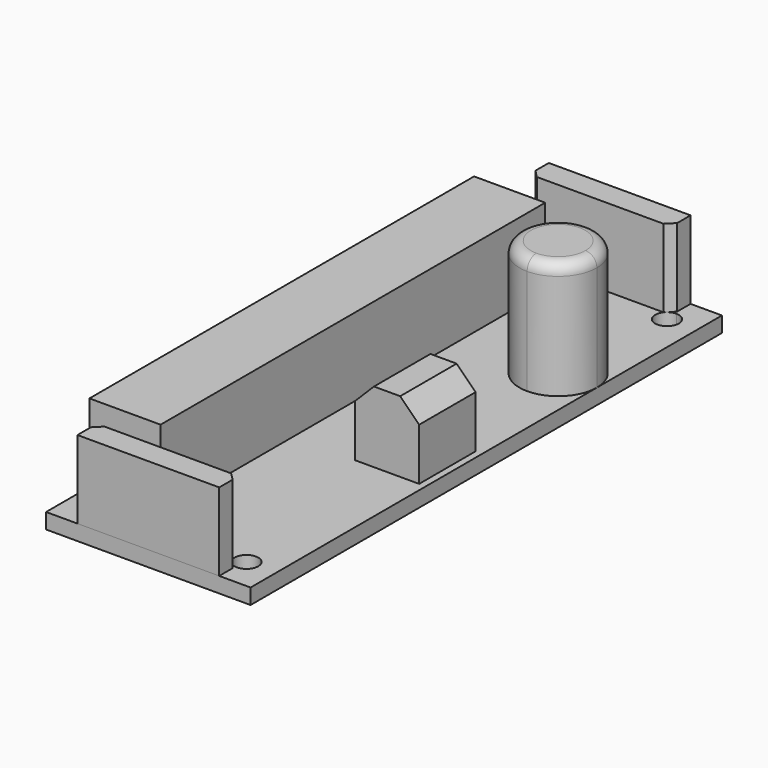
from build123d import *

# Parameters (mm, degrees)
F0_W       = 21.59
F0_H       = 62.21
F1_DEPTH   = 1.63
F4_DEPTH   = 12.34
F5_DEPTH   = 7.5
F2_R       = 1.25
F6_DEPTH   = 25
F7_SIZE    = 2
F8_R       = 1.2071067812
F10_DEPTH  = 8.23
F12_DEPTH  = 8.23
F13_SIZE   = 0.8
F13_2_SIZE = 0.8


with BuildPart() as f1:
    # F0 (on Top) → F1 (new body)
    with BuildSketch(Plane.XY):
        Rectangle(F0_W, F0_H)
    extrude(amount=F1_DEPTH)

    # F2 (on face) → F6 (cut)
    with BuildSketch(Plane.XY.offset(1.63)):
        with BuildLine():
            ThreePointArc((7.675, 29.005), (6.7911165235, 26.8711165235), (8.925, 27.755))
            Line((8.925, 27.755), (7.675, 27.755))
            Line((7.675, 27.755), (7.675, 29.005))
        make_face()
        with BuildLine():
            Line((7.675, 27.755), (8.925, 27.755))
            ThreePointArc((8.925, 27.755), (8.5588834765, 28.6388834765), (7.675, 29.005))
            Line((7.675, 29.005), (7.675, 27.755))
        make_face()
        with Locations((-7.675, 27.755)):
            Circle(F2_R)
        with Locations((-7.675, -27.755)):
            Circle(F2_R)
        with Locations((7.675, -27.755)):
            Circle(F2_R)
    extrude(amount=-F6_DEPTH, mode=Mode.SUBTRACT)


with BuildPart() as f4:
    # F3 (on face) → F4 (new body)
    with BuildSketch(Plane.XY.offset(1.63)):
        with BuildLine():
            ThreePointArc((10.7950629295, 14.605), (9.5971296646, 17.4970667351), (6.7050629295, 18.695))
            ThreePointArc((6.7050629295, 18.695), (2.6150629295, 14.605), (6.7050629295, 10.515))
            ThreePointArc((6.7050629295, 10.515), (9.5971296646, 11.7129332649), (10.7950629295, 14.605))
        make_face()
    extrude(amount=F4_DEPTH)

    # F8
    f8_edges = [f4.edges().sort_by_distance(p)[0] for p in [
        (6.705063, 18.695, 13.97),
    ]]
    fillet(f8_edges, radius=F8_R)


with BuildPart() as f5:
    # F3 (on face) → F5 (new body)
    with BuildSketch(Plane.XY.offset(1.63)):
        Polygon((10.0900629295, -0.525), (6.7050629295, -0.525), (3.3200629295, -0.525), (3.3200629295, -7.975), (10.0900629295, -7.975), align=None)
    extrude(amount=F5_DEPTH)

    # F7
    f7_edges = [f5.edges().sort_by_distance(p)[0] for p in [
        (3.320063, -4.25, 9.13),
        (10.090063, -4.25, 9.13),
    ]]
    chamfer(f7_edges, length=F7_SIZE)


with BuildPart() as f10:
    # F9 (on face) → F10 (new body)
    with BuildSketch(Plane.XY.offset(1.63)):
        Polygon((-10.795, 25.38), (-10.795, 0), (-10.795, -25.38), (-3.285, -25.38), (-3.285, 25.38), align=None)
    extrude(amount=F10_DEPTH)


with BuildPart() as f12:
    # F11 (on face) → F12 (new body)
    with BuildSketch(Plane.XY.offset(1.63)):
        with BuildLine():
            Line((7.485, 31.105), (0, 31.105))
            Line((0, 31.105), (-7.485, 31.105))
            Line((-7.485, 31.105), (-7.485, 28.9904756169))
            ThreePointArc((-7.485, 28.9904756169), (-7.0487343616, 28.8368000509), (-6.6982195743, 28.535))
            Line((-6.6982195743, 28.535), (6.6982195743, 28.535))
            ThreePointArc((6.6982195743, 28.535), (7.0487343616, 28.8368000509), (7.485, 28.9904756169))
            Line((7.485, 28.9904756169), (7.485, 31.105))
        make_face()
        with BuildLine():
            Line((7.485, 28.535), (7.485, 28.9904756169))
            ThreePointArc((7.485, 28.9904756169), (7.0487343616, 28.8368000509), (6.6982195743, 28.535))
            Line((6.6982195743, 28.535), (7.485, 28.535))
        make_face()
        with BuildLine():
            ThreePointArc((-6.6982195743, 28.535), (-7.0487343616, 28.8368000509), (-7.485, 28.9904756169))
            Line((-7.485, 28.9904756169), (-7.485, 28.535))
            Line((-7.485, 28.535), (-6.6982195743, 28.535))
        make_face()
    extrude(amount=F12_DEPTH)

    # F13
    f13_edges = [f12.edges().sort_by_distance(p)[0] for p in [
        (-7.485, 28.535, 5.745),
        (7.485, 28.535, 5.745),
    ]]
    chamfer(f13_edges, length=F13_SIZE)


with BuildPart() as f12b:
    # F11 (on face) → F12, piece 2 (new body)
    with BuildSketch(Plane.XY.offset(1.63)):
        with BuildLine():
            Line((-7.485, -28.9904756169), (-7.485, -31.105))
            Line((-7.485, -31.105), (0, -31.105))
            Line((0, -31.105), (7.485, -31.105))
            Line((7.485, -31.105), (7.485, -28.9904756169))
            ThreePointArc((7.485, -28.9904756169), (7.0487343616, -28.8368000509), (6.6982195743, -28.535))
            Line((6.6982195743, -28.535), (-6.6982195743, -28.535))
            ThreePointArc((-6.6982195743, -28.535), (-7.0487343616, -28.8368000509), (-7.485, -28.9904756169))
        make_face()
        with BuildLine():
            ThreePointArc((6.6982195743, -28.535), (7.0487343616, -28.8368000509), (7.485, -28.9904756169))
            Line((7.485, -28.9904756169), (7.485, -28.535))
            Line((7.485, -28.535), (6.6982195743, -28.535))
        make_face()
        with BuildLine():
            Line((-7.485, -28.535), (-7.485, -28.9904756169))
            ThreePointArc((-7.485, -28.9904756169), (-7.0487343616, -28.8368000509), (-6.6982195743, -28.535))
            Line((-6.6982195743, -28.535), (-7.485, -28.535))
        make_face()
    extrude(amount=F12_DEPTH)

    # F13#2
    f13_2_edges = [f12b.edges().sort_by_distance(p)[0] for p in [
        (-7.485, -28.535, 5.745),
        (7.485, -28.535, 5.745),
    ]]
    chamfer(f13_2_edges, length=F13_2_SIZE)


solid = Compound([f1.part, f4.part, f5.part, f10.part, f12.part, f12b.part])
